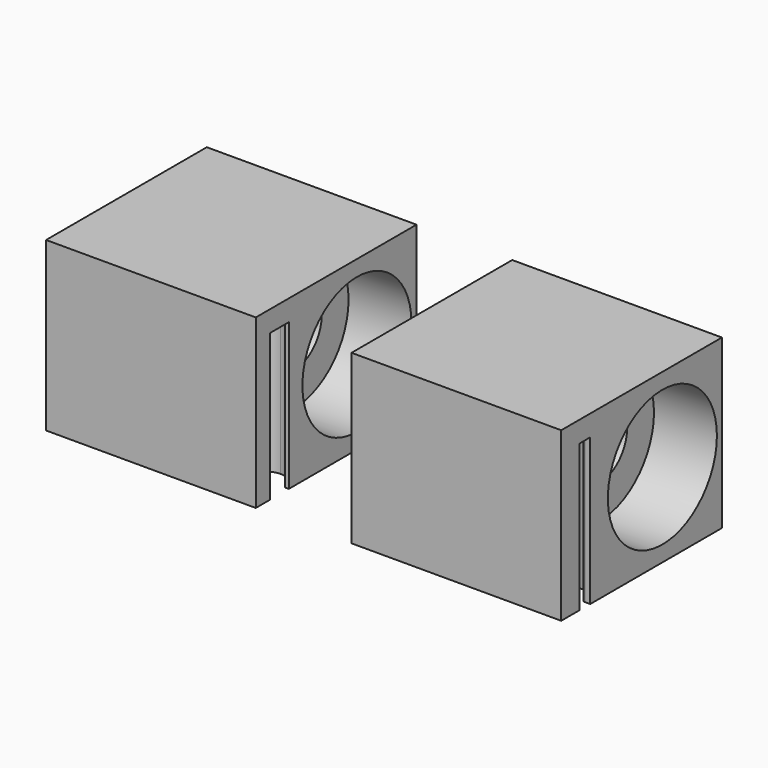
from build123d import *

# Parameters (mm, degrees)
F1_DEPTH       = 1
F2_DEPTH       = 7
F4_D           = 3.3
F4_CBORE_D     = 6.5
F4_CBORE_DEPTH = 3
F6_D           = 3.3
F6_CBORE_D     = 6.5
F6_CBORE_DEPTH = 3


# Not quite as in the source:
# - a feature names something its author has since deleted; it is built from what else it names


with BuildPart() as f1:
    # F0 (on Top) → F1 (new body)
    with BuildSketch(Plane.XY):
        with BuildLine():
            ThreePointArc((-32.9779816215, 23.288556752), (-32.6838322098, 23.2041958107), (-32.479105217, 22.9767589991))
            ThreePointArc((-32.479105217, 22.9767589991), (-32.4203699072, 22.8266189059), (-32.3865247301, 22.6689915346))
            ThreePointArc((-32.3865247301, 22.6689915346), (-32.3367132674, 22.5757853402), (-32.2378061964, 22.538556752))
            Line((-32.2378061964, 22.538556752), (-31.9779816215, 22.538556752))
            Line((-31.9779816215, 22.538556752), (-31.7181570466, 22.538556752))
            ThreePointArc((-31.7181570466, 22.538556752), (-31.6192499756, 22.5757853402), (-31.5694385129, 22.6689915346))
            ThreePointArc((-31.5694385129, 22.6689915346), (-31.5355933359, 22.8266189059), (-31.476858026, 22.9767589991))
            ThreePointArc((-31.476858026, 22.9767589991), (-31.2721310332, 23.2041958107), (-30.9779816215, 23.288556752))
            ThreePointArc((-30.9779816215, 23.288556752), (-30.6838322098, 23.2041958107), (-30.479105217, 22.9767589991))
            ThreePointArc((-30.479105217, 22.9767589991), (-30.4203699072, 22.8266189059), (-30.3865247301, 22.6689915346))
            ThreePointArc((-30.3865247301, 22.6689915346), (-30.3367132674, 22.5757853402), (-30.2378061964, 22.538556752))
            Line((-30.2378061964, 22.538556752), (-29.9779816215, 22.538556752))
            Line((-29.9779816215, 22.538556752), (-29.7181570466, 22.538556752))
            ThreePointArc((-29.7181570466, 22.538556752), (-29.6192499756, 22.5757853402), (-29.5694385129, 22.6689915346))
            ThreePointArc((-29.5694385129, 22.6689915346), (-29.5355933359, 22.8266189059), (-29.476858026, 22.9767589991))
            ThreePointArc((-29.476858026, 22.9767589991), (-29.2721310332, 23.2041958107), (-28.9779816215, 23.288556752))
            ThreePointArc((-28.9779816215, 23.288556752), (-28.6838322098, 23.2041958107), (-28.479105217, 22.9767589991))
            ThreePointArc((-28.479105217, 22.9767589991), (-28.4203699072, 22.8266189059), (-28.3865247301, 22.6689915346))
            ThreePointArc((-28.3865247301, 22.6689915346), (-28.3367132674, 22.5757853402), (-28.2378061964, 22.538556752))
            Line((-28.2378061964, 22.538556752), (-27.9779816215, 22.538556752))
            Line((-27.9779816215, 22.538556752), (-27.7181570466, 22.538556752))
            ThreePointArc((-27.7181570466, 22.538556752), (-27.6192499756, 22.5757853402), (-27.5694385129, 22.6689915346))
            ThreePointArc((-27.5694385129, 22.6689915346), (-27.5355933359, 22.8266189059), (-27.476858026, 22.9767589991))
            ThreePointArc((-27.476858026, 22.9767589991), (-27.2721310332, 23.2041958107), (-26.9779816215, 23.288556752))
            ThreePointArc((-26.9779816215, 23.288556752), (-26.6838322098, 23.2041958107), (-26.479105217, 22.9767589991))
            ThreePointArc((-26.479105217, 22.9767589991), (-26.4203699072, 22.8266189059), (-26.3865247301, 22.6689915346))
            ThreePointArc((-26.3865247301, 22.6689915346), (-26.3367132674, 22.5757853402), (-26.2378061964, 22.538556752))
            Line((-26.2378061964, 22.538556752), (-25.9779816215, 22.538556752))
            Line((-25.9779816215, 22.538556752), (-25.7181570466, 22.538556752))
            ThreePointArc((-25.7181570466, 22.538556752), (-25.6192499756, 22.5757853402), (-25.5694385129, 22.6689915346))
            ThreePointArc((-25.5694385129, 22.6689915346), (-25.5355933359, 22.8266189059), (-25.476858026, 22.9767589991))
            ThreePointArc((-25.476858026, 22.9767589991), (-25.2721310332, 23.2041958107), (-24.9779816215, 23.288556752))
            ThreePointArc((-24.9779816215, 23.288556752), (-24.6838322098, 23.2041958107), (-24.479105217, 22.9767589991))
            ThreePointArc((-24.479105217, 22.9767589991), (-24.4203699072, 22.8266189059), (-24.3865247301, 22.6689915346))
            ThreePointArc((-24.3865247301, 22.6689915346), (-24.3367132674, 22.5757853402), (-24.2378061964, 22.538556752))
            Line((-24.2378061964, 22.538556752), (-23.9779816215, 22.538556752))
            Line((-23.9779816215, 22.538556752), (-23.9779816215, 30.388556752))
            Line((-23.9779816215, 30.388556752), (-33.9779816215, 30.388556752))
            Line((-33.9779816215, 30.388556752), (-33.9779816215, 22.538556752))
            Line((-33.9779816215, 22.538556752), (-33.7181570466, 22.538556752))
            ThreePointArc((-33.7181570466, 22.538556752), (-33.6192499756, 22.5757853402), (-33.5694385129, 22.6689915346))
            ThreePointArc((-33.5694385129, 22.6689915346), (-33.5355933359, 22.8266189059), (-33.476858026, 22.9767589991))
            ThreePointArc((-33.476858026, 22.9767589991), (-33.2721310332, 23.2041958107), (-32.9779816215, 23.288556752))
        make_face()
        with BuildLine():
            ThreePointArc((-32.3865247301, 22.6689915346), (-32.4203699072, 22.8266189059), (-32.479105217, 22.9767589991))
            ThreePointArc((-32.479105217, 22.9767589991), (-32.6838322098, 23.2041958107), (-32.9779816215, 23.288556752))
            ThreePointArc((-32.9779816215, 23.288556752), (-33.2721310332, 23.2041958107), (-33.476858026, 22.9767589991))
            ThreePointArc((-33.476858026, 22.9767589991), (-33.5355933359, 22.8266189059), (-33.5694385129, 22.6689915346))
            ThreePointArc((-33.5694385129, 22.6689915346), (-33.6192499756, 22.5757853402), (-33.7181570466, 22.538556752))
            Line((-33.7181570466, 22.538556752), (-33.9779816215, 22.538556752))
            Line((-33.9779816215, 22.538556752), (-33.9779816215, 21.908556752))
            Line((-33.9779816215, 21.908556752), (-31.9779816215, 21.908556752))
            Line((-31.9779816215, 21.908556752), (-29.9779816215, 21.908556752))
            Line((-29.9779816215, 21.908556752), (-27.9779816215, 21.908556752))
            Line((-27.9779816215, 21.908556752), (-25.9779816215, 21.908556752))
            Line((-25.9779816215, 21.908556752), (-23.9779816215, 21.908556752))
            Line((-23.9779816215, 21.908556752), (-23.9779816215, 22.538556752))
            Line((-23.9779816215, 22.538556752), (-24.2378061964, 22.538556752))
            ThreePointArc((-24.2378061964, 22.538556752), (-24.3367132674, 22.5757853402), (-24.3865247301, 22.6689915346))
            ThreePointArc((-24.3865247301, 22.6689915346), (-24.4203699072, 22.8266189059), (-24.479105217, 22.9767589991))
            ThreePointArc((-24.479105217, 22.9767589991), (-24.6838322098, 23.2041958107), (-24.9779816215, 23.288556752))
            ThreePointArc((-24.9779816215, 23.288556752), (-25.2721310332, 23.2041958107), (-25.476858026, 22.9767589991))
            ThreePointArc((-25.476858026, 22.9767589991), (-25.5355933359, 22.8266189059), (-25.5694385129, 22.6689915346))
            ThreePointArc((-25.5694385129, 22.6689915346), (-25.6192499756, 22.5757853402), (-25.7181570466, 22.538556752))
            Line((-25.7181570466, 22.538556752), (-25.9779816215, 22.538556752))
            Line((-25.9779816215, 22.538556752), (-26.2378061964, 22.538556752))
            ThreePointArc((-26.2378061964, 22.538556752), (-26.3367132674, 22.5757853402), (-26.3865247301, 22.6689915346))
            ThreePointArc((-26.3865247301, 22.6689915346), (-26.4203699072, 22.8266189059), (-26.479105217, 22.9767589991))
            ThreePointArc((-26.479105217, 22.9767589991), (-26.6838322098, 23.2041958107), (-26.9779816215, 23.288556752))
            ThreePointArc((-26.9779816215, 23.288556752), (-27.2721310332, 23.2041958107), (-27.476858026, 22.9767589991))
            ThreePointArc((-27.476858026, 22.9767589991), (-27.5355933359, 22.8266189059), (-27.5694385129, 22.6689915346))
            ThreePointArc((-27.5694385129, 22.6689915346), (-27.6192499756, 22.5757853402), (-27.7181570466, 22.538556752))
            Line((-27.7181570466, 22.538556752), (-27.9779816215, 22.538556752))
            Line((-27.9779816215, 22.538556752), (-28.2378061964, 22.538556752))
            ThreePointArc((-28.2378061964, 22.538556752), (-28.3367132674, 22.5757853402), (-28.3865247301, 22.6689915346))
            ThreePointArc((-28.3865247301, 22.6689915346), (-28.4203699072, 22.8266189059), (-28.479105217, 22.9767589991))
            ThreePointArc((-28.479105217, 22.9767589991), (-28.6838322098, 23.2041958107), (-28.9779816215, 23.288556752))
            ThreePointArc((-28.9779816215, 23.288556752), (-29.2721310332, 23.2041958107), (-29.476858026, 22.9767589991))
            ThreePointArc((-29.476858026, 22.9767589991), (-29.5355933359, 22.8266189059), (-29.5694385129, 22.6689915346))
            ThreePointArc((-29.5694385129, 22.6689915346), (-29.6192499756, 22.5757853402), (-29.7181570466, 22.538556752))
            Line((-29.7181570466, 22.538556752), (-29.9779816215, 22.538556752))
            Line((-29.9779816215, 22.538556752), (-30.2378061964, 22.538556752))
            ThreePointArc((-30.2378061964, 22.538556752), (-30.3367132674, 22.5757853402), (-30.3865247301, 22.6689915346))
            ThreePointArc((-30.3865247301, 22.6689915346), (-30.4203699072, 22.8266189059), (-30.479105217, 22.9767589991))
            ThreePointArc((-30.479105217, 22.9767589991), (-30.6838322098, 23.2041958107), (-30.9779816215, 23.288556752))
            ThreePointArc((-30.9779816215, 23.288556752), (-31.2721310332, 23.2041958107), (-31.476858026, 22.9767589991))
            ThreePointArc((-31.476858026, 22.9767589991), (-31.5355933359, 22.8266189059), (-31.5694385129, 22.6689915346))
            ThreePointArc((-31.5694385129, 22.6689915346), (-31.6192499756, 22.5757853402), (-31.7181570466, 22.538556752))
            Line((-31.7181570466, 22.538556752), (-31.9779816215, 22.538556752))
            Line((-31.9779816215, 22.538556752), (-32.2378061964, 22.538556752))
            ThreePointArc((-32.2378061964, 22.538556752), (-32.3367132674, 22.5757853402), (-32.3865247301, 22.6689915346))
        make_face()
        Polygon((-31.9779816215, 21.908556752), (-33.9779816215, 21.908556752), (-33.9779816215, 20.808556752), (-23.9779816215, 20.808556752), (-23.9779816215, 21.908556752), (-25.9779816215, 21.908556752), (-27.9779816215, 21.908556752), (-29.9779816215, 21.908556752), align=None)
    extrude(amount=F1_DEPTH)

    # F0 (on Top) → F2 (join)
    with BuildSketch(Plane.XY):
        with BuildLine():
            ThreePointArc((-32.9779816215, 23.288556752), (-32.6838322098, 23.2041958107), (-32.479105217, 22.9767589991))
            ThreePointArc((-32.479105217, 22.9767589991), (-32.4203699072, 22.8266189059), (-32.3865247301, 22.6689915346))
            ThreePointArc((-32.3865247301, 22.6689915346), (-32.3367132674, 22.5757853402), (-32.2378061964, 22.538556752))
            Line((-32.2378061964, 22.538556752), (-31.9779816215, 22.538556752))
            Line((-31.9779816215, 22.538556752), (-31.7181570466, 22.538556752))
            ThreePointArc((-31.7181570466, 22.538556752), (-31.6192499756, 22.5757853402), (-31.5694385129, 22.6689915346))
            ThreePointArc((-31.5694385129, 22.6689915346), (-31.5355933359, 22.8266189059), (-31.476858026, 22.9767589991))
            ThreePointArc((-31.476858026, 22.9767589991), (-31.2721310332, 23.2041958107), (-30.9779816215, 23.288556752))
            ThreePointArc((-30.9779816215, 23.288556752), (-30.6838322098, 23.2041958107), (-30.479105217, 22.9767589991))
            ThreePointArc((-30.479105217, 22.9767589991), (-30.4203699072, 22.8266189059), (-30.3865247301, 22.6689915346))
            ThreePointArc((-30.3865247301, 22.6689915346), (-30.3367132674, 22.5757853402), (-30.2378061964, 22.538556752))
            Line((-30.2378061964, 22.538556752), (-29.9779816215, 22.538556752))
            Line((-29.9779816215, 22.538556752), (-29.7181570466, 22.538556752))
            ThreePointArc((-29.7181570466, 22.538556752), (-29.6192499756, 22.5757853402), (-29.5694385129, 22.6689915346))
            ThreePointArc((-29.5694385129, 22.6689915346), (-29.5355933359, 22.8266189059), (-29.476858026, 22.9767589991))
            ThreePointArc((-29.476858026, 22.9767589991), (-29.2721310332, 23.2041958107), (-28.9779816215, 23.288556752))
            ThreePointArc((-28.9779816215, 23.288556752), (-28.6838322098, 23.2041958107), (-28.479105217, 22.9767589991))
            ThreePointArc((-28.479105217, 22.9767589991), (-28.4203699072, 22.8266189059), (-28.3865247301, 22.6689915346))
            ThreePointArc((-28.3865247301, 22.6689915346), (-28.3367132674, 22.5757853402), (-28.2378061964, 22.538556752))
            Line((-28.2378061964, 22.538556752), (-27.9779816215, 22.538556752))
            Line((-27.9779816215, 22.538556752), (-27.7181570466, 22.538556752))
            ThreePointArc((-27.7181570466, 22.538556752), (-27.6192499756, 22.5757853402), (-27.5694385129, 22.6689915346))
            ThreePointArc((-27.5694385129, 22.6689915346), (-27.5355933359, 22.8266189059), (-27.476858026, 22.9767589991))
            ThreePointArc((-27.476858026, 22.9767589991), (-27.2721310332, 23.2041958107), (-26.9779816215, 23.288556752))
            ThreePointArc((-26.9779816215, 23.288556752), (-26.6838322098, 23.2041958107), (-26.479105217, 22.9767589991))
            ThreePointArc((-26.479105217, 22.9767589991), (-26.4203699072, 22.8266189059), (-26.3865247301, 22.6689915346))
            ThreePointArc((-26.3865247301, 22.6689915346), (-26.3367132674, 22.5757853402), (-26.2378061964, 22.538556752))
            Line((-26.2378061964, 22.538556752), (-25.9779816215, 22.538556752))
            Line((-25.9779816215, 22.538556752), (-25.7181570466, 22.538556752))
            ThreePointArc((-25.7181570466, 22.538556752), (-25.6192499756, 22.5757853402), (-25.5694385129, 22.6689915346))
            ThreePointArc((-25.5694385129, 22.6689915346), (-25.5355933359, 22.8266189059), (-25.476858026, 22.9767589991))
            ThreePointArc((-25.476858026, 22.9767589991), (-25.2721310332, 23.2041958107), (-24.9779816215, 23.288556752))
            ThreePointArc((-24.9779816215, 23.288556752), (-24.6838322098, 23.2041958107), (-24.479105217, 22.9767589991))
            ThreePointArc((-24.479105217, 22.9767589991), (-24.4203699072, 22.8266189059), (-24.3865247301, 22.6689915346))
            ThreePointArc((-24.3865247301, 22.6689915346), (-24.3367132674, 22.5757853402), (-24.2378061964, 22.538556752))
            Line((-24.2378061964, 22.538556752), (-23.9779816215, 22.538556752))
            Line((-23.9779816215, 22.538556752), (-23.9779816215, 30.388556752))
            Line((-23.9779816215, 30.388556752), (-33.9779816215, 30.388556752))
            Line((-33.9779816215, 30.388556752), (-33.9779816215, 22.538556752))
            Line((-33.9779816215, 22.538556752), (-33.7181570466, 22.538556752))
            ThreePointArc((-33.7181570466, 22.538556752), (-33.6192499756, 22.5757853402), (-33.5694385129, 22.6689915346))
            ThreePointArc((-33.5694385129, 22.6689915346), (-33.5355933359, 22.8266189059), (-33.476858026, 22.9767589991))
            ThreePointArc((-33.476858026, 22.9767589991), (-33.2721310332, 23.2041958107), (-32.9779816215, 23.288556752))
        make_face()
        Polygon((-31.9779816215, 21.908556752), (-33.9779816215, 21.908556752), (-33.9779816215, 20.808556752), (-23.9779816215, 20.808556752), (-23.9779816215, 21.908556752), (-25.9779816215, 21.908556752), (-27.9779816215, 21.908556752), (-29.9779816215, 21.908556752), align=None)
    extrude(amount=-F2_DEPTH)

    # F4 (through all)
    with Locations(Plane.YZ.offset(-23.9779816215)):
        with Locations((26.838556752, -3)):
            CounterBoreHole(F4_D / 2, F4_CBORE_D / 2, F4_CBORE_DEPTH)


with BuildPart() as f1b:
    # F0 (on Top) → F1, piece 2 (new body)
    with BuildSketch(Plane.XY):
        with BuildLine():
            Line((-48.5437250639, 22.7785576135), (-48.5437250639, 21.668556752))
            Line((-48.5437250639, 21.668556752), (-46.5437250639, 21.668556752))
            Line((-46.5437250639, 21.668556752), (-44.5437250639, 21.668556752))
            Line((-44.5437250639, 21.668556752), (-42.5437250639, 21.668556752))
            Line((-42.5437250639, 21.668556752), (-40.5437250639, 21.668556752))
            Line((-40.5437250639, 21.668556752), (-38.5437250639, 21.668556752))
            Line((-38.5437250639, 21.668556752), (-38.5437250639, 22.7785576135))
            Line((-38.5437250639, 22.7785576135), (-38.7271718496, 22.7785576135))
            ThreePointArc((-38.7271718496, 22.7785576135), (-38.7683162105, 22.9335455669), (-38.8291175479, 23.081927916))
            ThreePointArc((-38.8291175479, 23.081927916), (-39.1223754499, 23.4077161342), (-39.5437250639, 23.5285576135))
            ThreePointArc((-39.5437250639, 23.5285576135), (-39.9650746778, 23.4077161342), (-40.2583325799, 23.081927916))
            ThreePointArc((-40.2583325799, 23.081927916), (-40.3191339173, 22.9335455669), (-40.3602782781, 22.7785576135))
            Line((-40.3602782781, 22.7785576135), (-40.5437250639, 22.7785576135))
            Line((-40.5437250639, 22.7785576135), (-40.7271718496, 22.7785576135))
            ThreePointArc((-40.7271718496, 22.7785576135), (-40.7683162105, 22.9335455669), (-40.8291175479, 23.081927916))
            ThreePointArc((-40.8291175479, 23.081927916), (-41.1223754499, 23.4077161342), (-41.5437250639, 23.5285576135))
            ThreePointArc((-41.5437250639, 23.5285576135), (-41.9650746778, 23.4077161342), (-42.2583325799, 23.081927916))
            ThreePointArc((-42.2583325799, 23.081927916), (-42.3191339173, 22.9335455669), (-42.3602782781, 22.7785576135))
            Line((-42.3602782781, 22.7785576135), (-42.5437250639, 22.7785576135))
            Line((-42.5437250639, 22.7785576135), (-42.7271718496, 22.7785576135))
            ThreePointArc((-42.7271718496, 22.7785576135), (-42.7683162105, 22.9335455669), (-42.8291175479, 23.081927916))
            ThreePointArc((-42.8291175479, 23.081927916), (-43.1223754499, 23.4077161342), (-43.5437250639, 23.5285576135))
            ThreePointArc((-43.5437250639, 23.5285576135), (-43.9650746778, 23.4077161342), (-44.2583325799, 23.081927916))
            ThreePointArc((-44.2583325799, 23.081927916), (-44.3191339173, 22.9335455669), (-44.3602782781, 22.7785576135))
            Line((-44.3602782781, 22.7785576135), (-44.5437250639, 22.7785576135))
            Line((-44.5437250639, 22.7785576135), (-44.7271718496, 22.7785576135))
            ThreePointArc((-44.7271718496, 22.7785576135), (-44.7683162105, 22.9335455669), (-44.8291175479, 23.081927916))
            ThreePointArc((-44.8291175479, 23.081927916), (-45.1223754499, 23.4077161342), (-45.5437250639, 23.5285576135))
            ThreePointArc((-45.5437250639, 23.5285576135), (-45.9650746778, 23.4077161342), (-46.2583325799, 23.081927916))
            ThreePointArc((-46.2583325799, 23.081927916), (-46.3191339173, 22.9335455669), (-46.3602782781, 22.7785576135))
            Line((-46.3602782781, 22.7785576135), (-46.5437250639, 22.7785576135))
            Line((-46.5437250639, 22.7785576135), (-46.7271718496, 22.7785576135))
            ThreePointArc((-46.7271718496, 22.7785576135), (-46.7683162105, 22.9335455669), (-46.8291175479, 23.081927916))
            ThreePointArc((-46.8291175479, 23.081927916), (-47.1223754499, 23.4077161342), (-47.5437250639, 23.5285576135))
            ThreePointArc((-47.5437250639, 23.5285576135), (-47.9650746778, 23.4077161342), (-48.2583325799, 23.081927916))
            ThreePointArc((-48.2583325799, 23.081927916), (-48.3191339173, 22.9335455669), (-48.3602782781, 22.7785576135))
            Line((-48.3602782781, 22.7785576135), (-48.5437250639, 22.7785576135))
        make_face()
        Polygon((-46.5437250639, 21.668556752), (-48.5437250639, 21.668556752), (-48.5437250639, 20.808556752), (-38.5437250639, 20.808556752), (-38.5437250639, 21.668556752), (-40.5437250639, 21.668556752), (-42.5437250639, 21.668556752), (-44.5437250639, 21.668556752), align=None)
        with BuildLine():
            Line((-48.5437250639, 30.388556752), (-48.5437250639, 22.7785576135))
            Line((-48.5437250639, 22.7785576135), (-48.3602782781, 22.7785576135))
            ThreePointArc((-48.3602782781, 22.7785576135), (-48.3191339173, 22.9335455669), (-48.2583325799, 23.081927916))
            ThreePointArc((-48.2583325799, 23.081927916), (-47.9650746778, 23.4077161342), (-47.5437250639, 23.5285576135))
            ThreePointArc((-47.5437250639, 23.5285576135), (-47.1223754499, 23.4077161342), (-46.8291175479, 23.081927916))
            ThreePointArc((-46.8291175479, 23.081927916), (-46.7683162105, 22.9335455669), (-46.7271718496, 22.7785576135))
            Line((-46.7271718496, 22.7785576135), (-46.5437250639, 22.7785576135))
            Line((-46.5437250639, 22.7785576135), (-46.3602782781, 22.7785576135))
            ThreePointArc((-46.3602782781, 22.7785576135), (-46.3191339173, 22.9335455669), (-46.2583325799, 23.081927916))
            ThreePointArc((-46.2583325799, 23.081927916), (-45.9650746778, 23.4077161342), (-45.5437250639, 23.5285576135))
            ThreePointArc((-45.5437250639, 23.5285576135), (-45.1223754499, 23.4077161342), (-44.8291175479, 23.081927916))
            ThreePointArc((-44.8291175479, 23.081927916), (-44.7683162105, 22.9335455669), (-44.7271718496, 22.7785576135))
            Line((-44.7271718496, 22.7785576135), (-44.5437250639, 22.7785576135))
            Line((-44.5437250639, 22.7785576135), (-44.3602782781, 22.7785576135))
            ThreePointArc((-44.3602782781, 22.7785576135), (-44.3191339173, 22.9335455669), (-44.2583325799, 23.081927916))
            ThreePointArc((-44.2583325799, 23.081927916), (-43.9650746778, 23.4077161342), (-43.5437250639, 23.5285576135))
            ThreePointArc((-43.5437250639, 23.5285576135), (-43.1223754499, 23.4077161342), (-42.8291175479, 23.081927916))
            ThreePointArc((-42.8291175479, 23.081927916), (-42.7683162105, 22.9335455669), (-42.7271718496, 22.7785576135))
            Line((-42.7271718496, 22.7785576135), (-42.5437250639, 22.7785576135))
            Line((-42.5437250639, 22.7785576135), (-42.3602782781, 22.7785576135))
            ThreePointArc((-42.3602782781, 22.7785576135), (-42.3191339173, 22.9335455669), (-42.2583325799, 23.081927916))
            ThreePointArc((-42.2583325799, 23.081927916), (-41.9650746778, 23.4077161342), (-41.5437250639, 23.5285576135))
            ThreePointArc((-41.5437250639, 23.5285576135), (-41.1223754499, 23.4077161342), (-40.8291175479, 23.081927916))
            ThreePointArc((-40.8291175479, 23.081927916), (-40.7683162105, 22.9335455669), (-40.7271718496, 22.7785576135))
            Line((-40.7271718496, 22.7785576135), (-40.5437250639, 22.7785576135))
            Line((-40.5437250639, 22.7785576135), (-40.3602782781, 22.7785576135))
            ThreePointArc((-40.3602782781, 22.7785576135), (-40.3191339173, 22.9335455669), (-40.2583325799, 23.081927916))
            ThreePointArc((-40.2583325799, 23.081927916), (-39.9650746778, 23.4077161342), (-39.5437250639, 23.5285576135))
            ThreePointArc((-39.5437250639, 23.5285576135), (-39.1223754499, 23.4077161342), (-38.8291175479, 23.081927916))
            ThreePointArc((-38.8291175479, 23.081927916), (-38.7683162105, 22.9335455669), (-38.7271718496, 22.7785576135))
            Line((-38.7271718496, 22.7785576135), (-38.5437250639, 22.7785576135))
            Line((-38.5437250639, 22.7785576135), (-38.5437250639, 30.388556752))
            Line((-38.5437250639, 30.388556752), (-48.5437250639, 30.388556752))
        make_face()
    extrude(amount=F1_DEPTH)

    # F0 (on Top) → F2, piece 2 (join)
    with BuildSketch(Plane.XY):
        Polygon((-46.5437250639, 21.668556752), (-48.5437250639, 21.668556752), (-48.5437250639, 20.808556752), (-38.5437250639, 20.808556752), (-38.5437250639, 21.668556752), (-40.5437250639, 21.668556752), (-42.5437250639, 21.668556752), (-44.5437250639, 21.668556752), align=None)
        with BuildLine():
            Line((-48.5437250639, 30.388556752), (-48.5437250639, 22.7785576135))
            Line((-48.5437250639, 22.7785576135), (-48.3602782781, 22.7785576135))
            ThreePointArc((-48.3602782781, 22.7785576135), (-48.3191339173, 22.9335455669), (-48.2583325799, 23.081927916))
            ThreePointArc((-48.2583325799, 23.081927916), (-47.9650746778, 23.4077161342), (-47.5437250639, 23.5285576135))
            ThreePointArc((-47.5437250639, 23.5285576135), (-47.1223754499, 23.4077161342), (-46.8291175479, 23.081927916))
            ThreePointArc((-46.8291175479, 23.081927916), (-46.7683162105, 22.9335455669), (-46.7271718496, 22.7785576135))
            Line((-46.7271718496, 22.7785576135), (-46.5437250639, 22.7785576135))
            Line((-46.5437250639, 22.7785576135), (-46.3602782781, 22.7785576135))
            ThreePointArc((-46.3602782781, 22.7785576135), (-46.3191339173, 22.9335455669), (-46.2583325799, 23.081927916))
            ThreePointArc((-46.2583325799, 23.081927916), (-45.9650746778, 23.4077161342), (-45.5437250639, 23.5285576135))
            ThreePointArc((-45.5437250639, 23.5285576135), (-45.1223754499, 23.4077161342), (-44.8291175479, 23.081927916))
            ThreePointArc((-44.8291175479, 23.081927916), (-44.7683162105, 22.9335455669), (-44.7271718496, 22.7785576135))
            Line((-44.7271718496, 22.7785576135), (-44.5437250639, 22.7785576135))
            Line((-44.5437250639, 22.7785576135), (-44.3602782781, 22.7785576135))
            ThreePointArc((-44.3602782781, 22.7785576135), (-44.3191339173, 22.9335455669), (-44.2583325799, 23.081927916))
            ThreePointArc((-44.2583325799, 23.081927916), (-43.9650746778, 23.4077161342), (-43.5437250639, 23.5285576135))
            ThreePointArc((-43.5437250639, 23.5285576135), (-43.1223754499, 23.4077161342), (-42.8291175479, 23.081927916))
            ThreePointArc((-42.8291175479, 23.081927916), (-42.7683162105, 22.9335455669), (-42.7271718496, 22.7785576135))
            Line((-42.7271718496, 22.7785576135), (-42.5437250639, 22.7785576135))
            Line((-42.5437250639, 22.7785576135), (-42.3602782781, 22.7785576135))
            ThreePointArc((-42.3602782781, 22.7785576135), (-42.3191339173, 22.9335455669), (-42.2583325799, 23.081927916))
            ThreePointArc((-42.2583325799, 23.081927916), (-41.9650746778, 23.4077161342), (-41.5437250639, 23.5285576135))
            ThreePointArc((-41.5437250639, 23.5285576135), (-41.1223754499, 23.4077161342), (-40.8291175479, 23.081927916))
            ThreePointArc((-40.8291175479, 23.081927916), (-40.7683162105, 22.9335455669), (-40.7271718496, 22.7785576135))
            Line((-40.7271718496, 22.7785576135), (-40.5437250639, 22.7785576135))
            Line((-40.5437250639, 22.7785576135), (-40.3602782781, 22.7785576135))
            ThreePointArc((-40.3602782781, 22.7785576135), (-40.3191339173, 22.9335455669), (-40.2583325799, 23.081927916))
            ThreePointArc((-40.2583325799, 23.081927916), (-39.9650746778, 23.4077161342), (-39.5437250639, 23.5285576135))
            ThreePointArc((-39.5437250639, 23.5285576135), (-39.1223754499, 23.4077161342), (-38.8291175479, 23.081927916))
            ThreePointArc((-38.8291175479, 23.081927916), (-38.7683162105, 22.9335455669), (-38.7271718496, 22.7785576135))
            Line((-38.7271718496, 22.7785576135), (-38.5437250639, 22.7785576135))
            Line((-38.5437250639, 22.7785576135), (-38.5437250639, 30.388556752))
            Line((-38.5437250639, 30.388556752), (-48.5437250639, 30.388556752))
        make_face()
    extrude(amount=-F2_DEPTH)

    # F6 (through all)
    with Locations(Plane.YZ.offset(-38.5437250639)):
        with Locations((26.838556752, -3)):
            CounterBoreHole(F6_D / 2, F6_CBORE_D / 2, F6_CBORE_DEPTH)


solid = Compound([f1.part, f1b.part])
